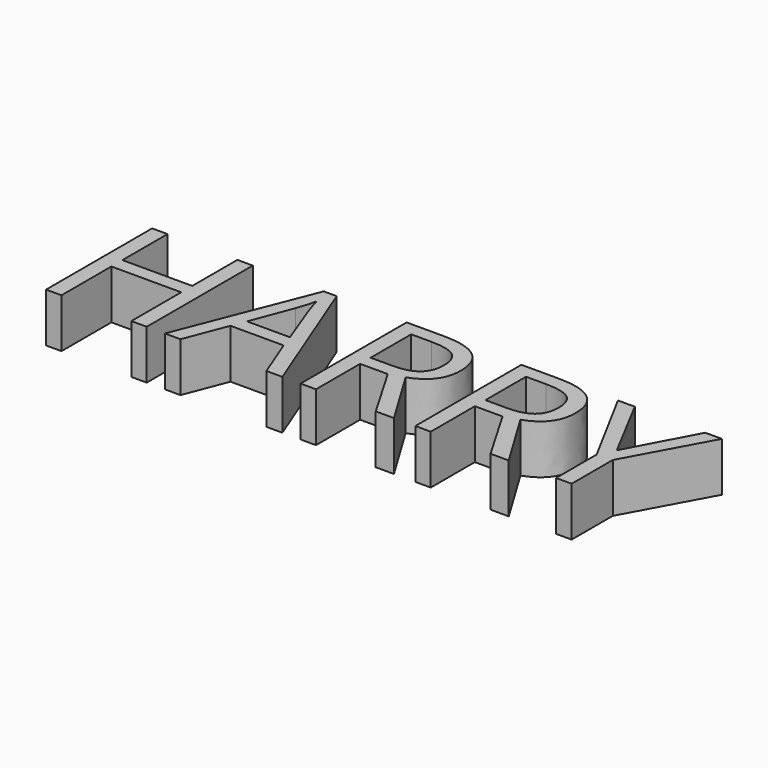
from build123d import *

# Parameters (mm, degrees)
F0_TEXT_SIZE = 38.3333225424
F1_DEPTH     = 10.16


# Not quite as in the source:
# - Text() gives the source's letters only with a copy of the font that has no kerning and outlines rounded to 1/6400 em; it was checked with that copy


with BuildPart() as f1:
    # F0 (on Top) → F1 (new body)
    with BuildSketch(Plane.XY):
        with Locations((-61.2931996584, -14.8315057158)):
            Text('HARRY', F0_TEXT_SIZE, font='Open Sans', text_align=(TextAlign.LEFT, TextAlign.BOTTOM))
    extrude(amount=F1_DEPTH)


solid = f1.part
